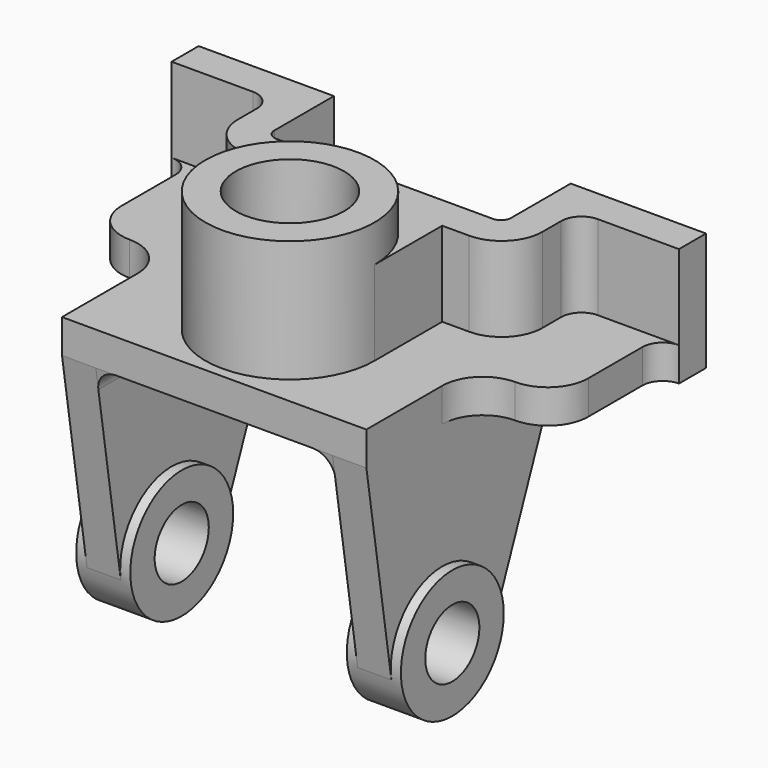
from build123d import *

# Parameters (mm, degrees)
F1_DEPTH      = 25
F0_R          = 16
F2_DEPTH      = 36
F4_DEPTH      = 10
F6_DEPTH      = 10
F8_R          = 19
F8_R_2        = 10
F9_DEPTH      = 8
F10_T4_DEPTH  = 103
F10_S6_R      = 25
F10_T7_DEPTH  = 53
F10_T11_DEPTH = 103
F10_S13_R     = 25
F10_T14_DEPTH = 53


# Not quite as in the source:
# - a fillet or chamfer that OpenCascade refuses, or shapes differently, is made with other operations: its cross-section is extruded or revolved along the edge and cut away or added
# - a pattern or mirror of a feature is missing from the dataset's text; its kind, count and spacing are read off the source's solid


with BuildPart() as f1:
    # F0 (on Top) → F1 (new body)
    with BuildSketch(Plane.XY):
        with BuildLine():
            Line((-35, 44), (-75, 44))
            Line((-75, 44), (-75, 34))
            Line((-75, 34), (-51, 34))
            ThreePointArc((-51, 34), (-46.7573593129, 32.2426406871), (-45, 28))
            Line((-45, 28), (-45, 21))
            ThreePointArc((-45, 21), (-41.4852813742, 12.5147186258), (-33, 9))
            Line((-33, 9), (-25, 9))
            Line((-25, 9), (-25, -16))
            ThreePointArc((-25, -16), (0, 9), (25, -16))
            Line((25, -16), (25, 9))
            Line((25, 9), (33, 9))
            ThreePointArc((33, 9), (41.4852813742, 12.5147186258), (45, 21))
            Line((45, 21), (45, 28))
            ThreePointArc((45, 28), (46.7573593129, 32.2426406871), (51, 34))
            Line((51, 34), (75, 34))
            Line((75, 34), (75, 44))
            Line((75, 44), (35, 44))
            Line((35, 44), (35, 34))
            Line((35, 34), (35, 22))
            ThreePointArc((35, 22), (34.1213203436, 19.8786796564), (32, 19))
            Line((32, 19), (-32, 19))
            ThreePointArc((-32, 19), (-34.1213203436, 19.8786796564), (-35, 22))
            Line((-35, 22), (-35, 34))
            Line((-35, 34), (-35, 44))
        make_face()
    extrude(amount=F1_DEPTH)

    # F0 (on Top) → F2 (join)
    with BuildSketch(Plane.XY):
        with BuildLine():
            ThreePointArc((25, -16), (0, 9), (-25, -16))
            ThreePointArc((-25, -16), (0, -41), (25, -16))
        make_face()
        with Locations((0, -16)):
            Circle(F0_R, mode=Mode.SUBTRACT)
    extrude(amount=F2_DEPTH)

    # F3 (on face) → F4 (join)
    with BuildSketch(Plane.XY):
        with BuildLine():
            Line((75, 34), (75, 44))
            Line((75, 44), (-75, 44))
            Line((-75, 44), (-75, 34))
            ThreePointArc((-75, 34), (-70.7573593129, 32.2426406871), (-69, 28))
            Line((-69, 28), (-69, 8))
            ThreePointArc((-69, 8), (-65.4852813742, -0.4852813742), (-57, -4))
            ThreePointArc((-57, -4), (-48.5147186258, -7.5147186258), (-45, -16))
            Line((-45, -16), (-45, -44))
            Line((-45, -44), (45, -44))
            Line((45, -44), (45, -16))
            ThreePointArc((45, -16), (48.5147186258, -7.5147186258), (57, -4))
            ThreePointArc((57, -4), (65.4852813742, -0.4852813742), (69, 8))
            Line((69, 8), (69, 28))
            ThreePointArc((69, 28), (70.7573593129, 32.2426406871), (75, 34))
        make_face()
    extrude(amount=-F4_DEPTH)

    # F5 (on face) → F6 (join)
    with BuildSketch(Plane.YZ.offset(45)):
        with BuildLine():
            ThreePointArc((-34.7712820587, -68.9392124579), (-17.4740489959, -47.0572657845), (3, -66))
            ThreePointArc((3, -66), (2.6502712249, -69.6286889144), (1.6139596592, -73.1237928888))
            Line((1.6139596592, -73.1237928888), (20.8237372905, -25.6265883042))
            ThreePointArc((20.8237372905, -25.6265883042), (30.0238648475, -14.2715739575), (44, -10))
            Line((44, -10), (34, -10))
            Line((34, -10), (-16, -10))
            Line((-16, -10), (-44, -10))
            Line((-44, -10), (-34.7712820587, -68.9392124579))
        make_face()
    f6 = extrude(amount=-F6_DEPTH)

    # F6_copies: F6 across plane
    add(f6.mirror(Plane(origin=(0, 0, 0), x_dir=(0, 0, -1), z_dir=(-1, 0, 0))))

    # F8 (on face) → F9 (join, symmetric)
    with BuildSketch(Plane.YZ.offset(40)):
        with Locations((-16, -66)):
            Circle(F8_R)
        with Locations((-16, -66)):
            Circle(F8_R_2, mode=Mode.SUBTRACT)
    f9 = extrude(amount=F9_DEPTH, both=True)

    # F9_copies: F9 across plane
    add(f9.mirror(Plane(origin=(0, 0, 0), x_dir=(0, 0, -1), z_dir=(-1, 0, 0))))

    # F10: fillet of radius 6 on 2 edges, made by hand


with BuildPart() as f10_tool2:
    # F10_s3 → F10_t4 (new body)
    with BuildSketch(Plane.XZ.offset(-44)):
        with BuildLine():
            ThreePointArc((29, -10), (33.2426406871, -11.7573593129), (35, -16))
            Line((35, -16), (35, -10))
            Line((35, -10), (29, -10))
        make_face()
    extrude(amount=F10_T4_DEPTH)

    split(bisect_by=Plane(origin=(0, -44.4753827877, -6.9639675517), x_dir=(1, 0, 0), z_dir=(0, 0.9879622136, 0.1546953925)), keep=Keep.TOP)

    # F10_s6 → F10_t7 (cut, symmetric)
    with BuildSketch(Plane.YZ.offset(32)):
        with Locations((44, -35)):
            Circle(F10_S6_R)
    extrude(amount=F10_T7_DEPTH, both=True, mode=Mode.SUBTRACT)


with BuildPart() as f1_1:
    add(f1.part)

    # F10_t1: union F10_tool2
    add(f10_tool2.part)


with BuildPart() as f10_tool9:
    # F10_s10 → F10_t11 (new body)
    with BuildSketch(Plane.XZ.offset(-44)):
        with BuildLine():
            ThreePointArc((-35, -16), (-33.2426406871, -11.7573593129), (-29, -10))
            Line((-29, -10), (-35, -10))
            Line((-35, -10), (-35, -16))
        make_face()
    extrude(amount=F10_T11_DEPTH)

    split(bisect_by=Plane(origin=(0, -44.4753827877, -6.9639675517), x_dir=(1, 0, 0), z_dir=(0, 0.9879622136, 0.1546953925)), keep=Keep.TOP)

    # F10_s13 → F10_t14 (cut, symmetric)
    with BuildSketch(Plane.YZ.offset(-32)):
        with Locations((44, -35)):
            Circle(F10_S13_R)
    extrude(amount=F10_T14_DEPTH, both=True, mode=Mode.SUBTRACT)


with BuildPart() as f1_2:
    add(f1_1.part)

    # F10_t8: union F10_tool9
    add(f10_tool9.part)


solid = f1_2.part
